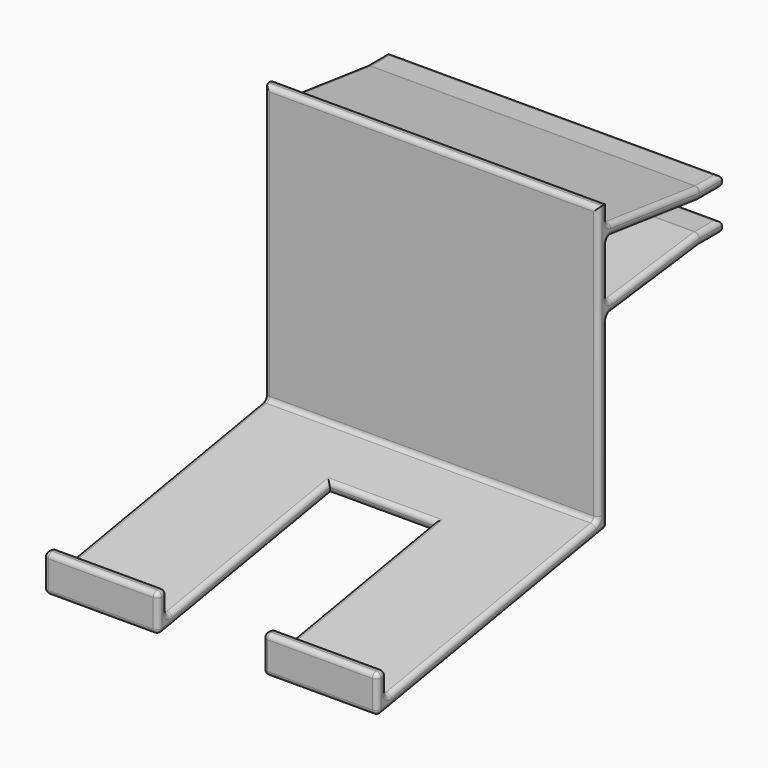
from build123d import *

# Parameters (mm, degrees)
F1_DEPTH = 17.5
F2_W     = 11
F2_H     = 3.4183796076
F2_H_2   = 21.5816203924
F3_DEPTH = 12.5
F4_F1_R  = 0.5
F4_F2_R  = 0.5


with BuildPart() as f1:
    # F0 (on Right) → F1 (new body, symmetric)
    with BuildSketch(Plane.YZ):
        Polygon((3.763121268, 2.5496664763), (-8.3115880299, 4.0590051386), (-8.3115880299, 6.0590051386), (-9.5115880299, 6.0590051386), (-9.5115880299, -22.9525872383), (-37.3115880299, -27.854477302), (-37.3115880299, -25.2660696788), (-38.5115880299, -25.2660696788), (-38.5115880299, -28.0660696788), (-38.5115880299, -29.2660696788), (-8.3115880299, -23.9409948614), (-8.3115880299, -4.3596721859), (3.763121268, -2.8503335237), (6.6884119701, -2.8503335237), (6.6884119701, -1.6503335237), (3.6884119701, -1.6503335237), (-8.3115880299, -3.1503335237), (-8.3115880299, 2.8496664763), (3.6884119701, 1.3496664763), (6.6884119701, 1.3496664763), (6.6884119701, 2.5496664763), align=None)
    extrude(amount=F1_DEPTH, both=True)

    # F2 (on face) → F3 (cut, symmetric)
    with BuildSketch(Plane(origin=(0, 3.6383141153, -20.6339046964), x_dir=(1, 0, 0), z_dir=(0, -0.1736481777, 0.984807753))):
        with Locations((0, -43.2908101962)):
            Rectangle(F2_W, F2_H)
        with Locations((0, -30.7908101962)):
            Rectangle(F2_W, F2_H_2)
    extrude(amount=F3_DEPTH, both=True, mode=Mode.SUBTRACT)

    # F4: fillet of radius 0.5 on 60 edges, made by hand

    # F4_f1
    f4_f1_edges = [f1.edges().sort_by_distance(p)[0] for p in [
        (0, -9.5115880299, -22.9525872383),
        (11.5, -37.3115880299, -27.854477302),
        (-11.5, -37.3115880299, -27.854477302),
        (0, -8.3115880299, -4.3596721859),
        (0, -8.3115880299, 4.0590051386),
        (0, 3.763121268, 2.5496664763),
        (0, 3.763121268, -2.8503335237),
        (0, -8.3115880299, 2.8496664763),
        (0, -8.3115880299, -3.1503335237),
    ]]
    fillet(f4_f1_edges, radius=F4_F1_R)

    # F4_f2
    f4_f2_edges = [f1.edges().sort_by_distance(p)[0] for p in [
        (0, -9.5115880299, 6.0590051386),
        (-17.5, -9.5115880299, -8.237016142),
        (17.5, -9.5115880299, -8.237016142),
        (17.5, -23.3247639411, -25.3882228407),
        (5.5, -26.391302443, -25.9289363159),
        (0, -16.0578409449, -24.1068682497),
        (-5.5, -26.391302443, -25.9289363159),
        (-17.5, -23.3247639411, -25.3882228407),
        (-11.5, -38.5115880299, -29.2660696788),
        (-17.5, -38.5115880299, -27.2660696788),
        (-11.5, -38.5115880299, -25.2660696788),
        (-5.5, -38.5115880299, -27.2660696788),
        (11.5, -38.5115880299, -29.2660696788),
        (5.5, -38.5115880299, -27.2660696788),
        (11.5, -38.5115880299, -25.2660696788),
        (17.5, -38.5115880299, -27.2660696788),
        (-11.5, -37.3115880299, -25.2660696788),
        (-5.5, -37.9115880299, -25.2660696788),
        (-17.5, -37.9115880299, -25.2660696788),
        (11.5, -37.3115880299, -25.2660696788),
        (17.5, -37.9115880299, -25.2660696788),
        (5.5, -37.9115880299, -25.2660696788),
        (-5.5, -27.1821084444, -27.2683767505),
        (0, -15.8526288589, -25.2706838222),
        (5.5, -27.1821084444, -27.2683767505),
        (17.5, -23.4115880299, -26.6035322701),
        (0, -8.3115880299, -23.9409948614),
        (-17.5, -23.4115880299, -26.6035322701),
        (-17.5, -8.3115880299, -14.3710290783),
        (17.5, -8.3115880299, -14.3710290783),
        (-17.5, -8.3115880299, 5.2797006932),
        (0, -8.3115880299, 6.0590051386),
        (17.5, -8.3115880299, 5.2797006932),
        (0, 6.6884119701, 2.5496664763),
        (-17.5, 5.2413310561, 2.5496664763),
        (17.5, 5.2413310561, 2.5496664763),
        (0, 3.6884119701, 1.3496664763),
        (-17.5, 5.1884119701, 1.3496664763),
        (0, 6.6884119701, 1.3496664763),
        (17.5, 5.1884119701, 1.3496664763),
        (-17.5, 5.2413310561, -2.8503335237),
        (0, 6.6884119701, -2.8503335237),
        (17.5, 5.2413310561, -2.8503335237),
        (0, 6.6884119701, -1.6503335237),
        (-17.5, 5.1884119701, -1.6503335237),
        (0, 3.6884119701, -1.6503335237),
        (17.5, 5.1884119701, -1.6503335237),
        (-17.5, -2.0305793463, 2.0645403909),
        (17.5, -2.0305793463, 2.0645403909),
        (-17.5, -2.0305793463, -2.3652074382),
        (17.5, -2.0305793463, -2.3652074382),
        (17.5, -8.1424893115, -2.9587815023),
        (-17.5, -8.1424893115, -2.9587815023),
        (17.5, -8.1424893115, 2.658114455),
        (-17.5, -8.1424893115, 2.658114455),
        (17.5, 3.7631814214, -2.8512997226),
        (-17.5, 3.7631814214, -2.8512997226),
        (17.5, 3.7631814214, 2.5506326753),
        (-17.5, 3.7631814214, 2.5506326753),
        (17.5, -8.1864271178, 4.1694949662),
        (-17.5, -8.1864271178, 4.1694949662),
        (17.5, -8.1864271178, -4.4701620135),
        (-17.5, -8.1864271178, -4.4701620135),
        (-17.5, -9.6285658084, -22.8544312275),
        (-17.5, -37.1329818348, -27.6416227272),
        (-5.5, -37.1329818348, -27.6416227272),
        (5.5, -37.1329818348, -27.6416227272),
        (17.5, -9.6285658084, -22.8544312275),
        (17.5, -37.1329818348, -27.6416227272),
    ]]
    fillet(f4_f2_edges, radius=F4_F2_R)


solid = f1.part
